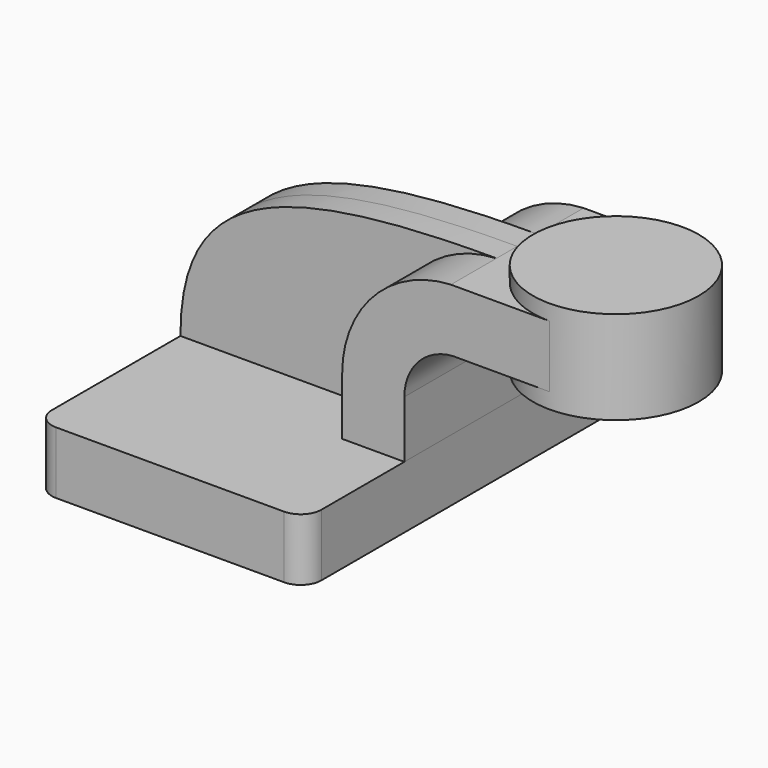
from build123d import *

# Parameters (mm, degrees)
F1_DEPTH = 63.5
F0_W     = 25.4
F0_H     = 19.05
F2_DEPTH = 25.4
F3_DEPTH = 7.9375
F5_R     = 6.35


# Not quite as in the source:
# - ends of sketch curves that miss each other by under 0.0002 mm in the source are joined


with BuildPart() as f1:
    # F0 (on Front) → F1 (new body, symmetric)
    with BuildSketch(Plane.XZ):
        Polygon((-41.275, 9.525), (-41.275, -9.525), (41.275, -9.525), (41.275, 9.525), (22.225, 9.525), align=None)
    extrude(amount=F1_DEPTH, both=True)

    # F5
    f5_edges = [f1.edges().sort_by_distance(p)[0] for p in [
        (41.275, -63.5, 0),
        (41.275, 63.5, 0),
        (-41.275, 63.5, 0),
        (-41.275, -63.5, 0),
    ]]
    fillet(f5_edges, radius=F5_R)


with BuildPart() as f2:
    # F0 (on Front) → F2 (new body, symmetric)
    with BuildSketch(Plane.XZ):
        with BuildLine():
            Line((22.225, 9.525), (41.275, 9.525))
            Line((41.275, 9.525), (41.275, 27.038495028))
            ThreePointArc((41.275, 27.038495028), (45.5416010852, 37.8671929938), (56.0480015287, 42.8752))
            Line((56.0480015287, 42.8752), (60.325, 42.8752))
            Line((60.325, 42.8752), (60.325, 61.9252))
            Line((60.325, 61.9252), (55.5149338856, 61.9252))
            ThreePointArc((55.5149338856, 61.9252), (31.8828245638, 51.1491870645), (22.225, 27.038495028))
            Line((22.225, 27.038495028), (22.225, 9.525))
        make_face()
        with Locations((73.025, 52.4002)):
            Rectangle(F0_W, F0_H)
    extrude(amount=F2_DEPTH, both=True)

    # F0 (on Front) → F4 (revolve)
    with BuildSketch(Plane.XZ):
        Polygon((85.725, 66.675), (85.725, 61.9252), (85.725, 42.8752), (85.725, 38.1), (111.125, 38.1), (111.125, 66.675), align=None)
    revolve(axis=Axis((85.725, 0, 52.3875), (0, 0, 1)))


with BuildPart() as f3:
    # F0 (on Front) → F3 (new body, symmetric)
    with BuildSketch(Plane.XZ):
        with BuildLine():
            add(Edge.make_bspline(
                [(-41.275, 9.525), (-41.275, 49.6220278599), (-13.2913665774, 61.9252), (55.5149338856, 61.9252)],
                knots=[0, 0, 0, 0, 110.0639462386, 110.0639462386, 110.0639462386, 110.0639462386], degree=3))
            Line((-41.275, 9.525), (22.225, 9.525))
            Line((22.225, 9.525), (22.225, 27.038495028))
            ThreePointArc((22.225, 27.038495028), (31.8828245638, 51.1491870645), (55.5149338856, 61.9252))
        make_face()
    extrude(amount=F3_DEPTH, both=True)


solid = Compound([f1.part, f2.part, f3.part])
